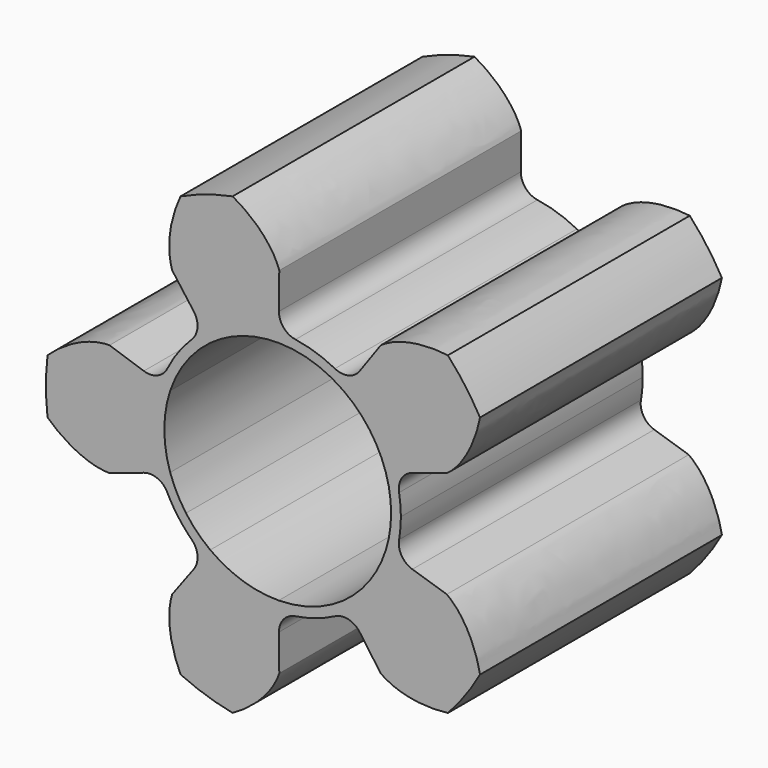
from build123d import *

# Parameters (mm, degrees)
F3_DEPTH        = 3.175
F3_COPIES_COUNT = 5
F4_R            = 0.2032


# Not quite as in the source:
# - a feature of the source that left no trace in its solid (it failed there, or was rolled back) is left out
# - a pattern or mirror of a feature is missing from the dataset's text; its kind, count and spacing are read off the source's solid


with BuildPart() as f3:
    # F2 (on Front) → F3 (new body)
    with BuildSketch(Plane.XZ):
        with BuildLine():
            add(Edge.make_bspline(
                [(-0.4736975711, 2.3876302001), (-0.3454827241, 2.306853053), (-0.3815948665, 2.3342231222), (-0.2290140547, 2.2185792667), (-0.1542942205, 2.1416333305), (-0.084040716, 2.0556874167), (-0.0391643261, 1.9888964707), (0.0044637369, 1.8978667818), (-0.0039604646, 1.9154438273), (0.0163220053, 1.8619585339)],
                knots=[0, 0, 0, 0, 0.1738109625, 0.3386813621, 0.4939363745, 0.6387860849, 0.7722773022, 0.8932124897, 1, 1, 1, 1], degree=3))
            ThreePointArc((-0.4736975711, 2.3876302001), (-0.7521988671, 2.3150300701), (-1.0201844344, 2.2100658545))
            add(Edge.make_bspline(
                [(-1.0201844344, 2.2100658545), (-1.0764328087, 2.0693529736), (-1.0633051948, 2.1127220094), (-1.1187719118, 1.929479414), (-1.133993841, 1.8233096274), (-1.1403123794, 1.7124839487), (-1.1373594084, 1.6320712581), (-1.1191493442, 1.5327827608), (-1.1226655501, 1.5519545107), (-1.1076365463, 1.4967622627)],
                knots=[0, 0, 0, 0, 0.1738109625, 0.3386813621, 0.4939363745, 0.6387860849, 0.7722773022, 0.8932124897, 1, 1, 1, 1], degree=3))
            Line((-1.1076365463, 1.4967622627), (-0.7690003409, 1.0391591847))
            ThreePointArc((-0.7690003409, 1.0391591847), (-0.399483007, 1.2294822742), (0.011331901, 1.2927044997))
            Line((0.011331901, 1.2927044997), (0.0163220053, 1.8619585339))
        make_face()
        with BuildLine():
            Line((0.0104366669, 1.1905792568), (0.011331901, 1.2927044997))
            ThreePointArc((0.011331901, 1.2927044997), (-0.399483007, 1.2294822742), (-0.7690003409, 1.0391591847))
            Line((-0.7690003409, 1.0391591847), (-0.7082483697, 0.957064333))
            ThreePointArc((-0.7082483697, 0.957064333), (-0.3679233589, 1.1323516647), (0.0104366669, 1.1905792568))
        make_face()
        with BuildLine():
            ThreePointArc((1.2927541667, 0), (0.9181129281, 0.9100999872), (0.011331901, 1.2927044997))
            Line((0.011331901, 1.2927044997), (0.0104366669, 1.1905792568))
            ThreePointArc((0.0104366669, 1.1905792568), (0.8455808794, 0.8382009706), (1.190625, 0))
            ThreePointArc((1.190625, 0), (-0.5358776332, -1.06321355), (-0.7082483697, 0.957064333))
            Line((-0.7082483697, 0.957064333), (-0.7690003409, 1.0391591847))
            ThreePointArc((-0.7690003409, 1.0391591847), (-0.5818440257, -1.1544136456), (1.2927541667, 0))
        make_face()
    extrude(amount=F3_DEPTH)

    # F3_copies: F3 ×5 about axis
    f3_copies_axis = Axis((0, 0, 0), (0, 1, 0))


with BuildPart() as f3_1:
    add(f3.part)
    for i in range(1, F3_COPIES_COUNT):
        add(f3.part.rotate(f3_copies_axis, i * 360 / F3_COPIES_COUNT))

    # F4
    f4_edges = [f3_1.edges().sort_by_distance(p)[0] for p in [
        (-1.225933, -1.5875, 0.410245),
        (-0.769, -1.5875, 1.039159),
        (-1.225933, -1.5875, -0.410245),
        (-0.769, -1.5875, -1.039159),
        (0.011332, -1.5875, -1.292704),
        (0.750665, -1.5875, -1.052481),
        (1.232937, -1.5875, -0.38869),
        (1.232937, -1.5875, 0.38869),
        (0.750665, -1.5875, 1.052481),
        (0.011332, -1.5875, 1.292704),
    ]]
    fillet(f4_edges, radius=F4_R)


solid = f3_1.part
